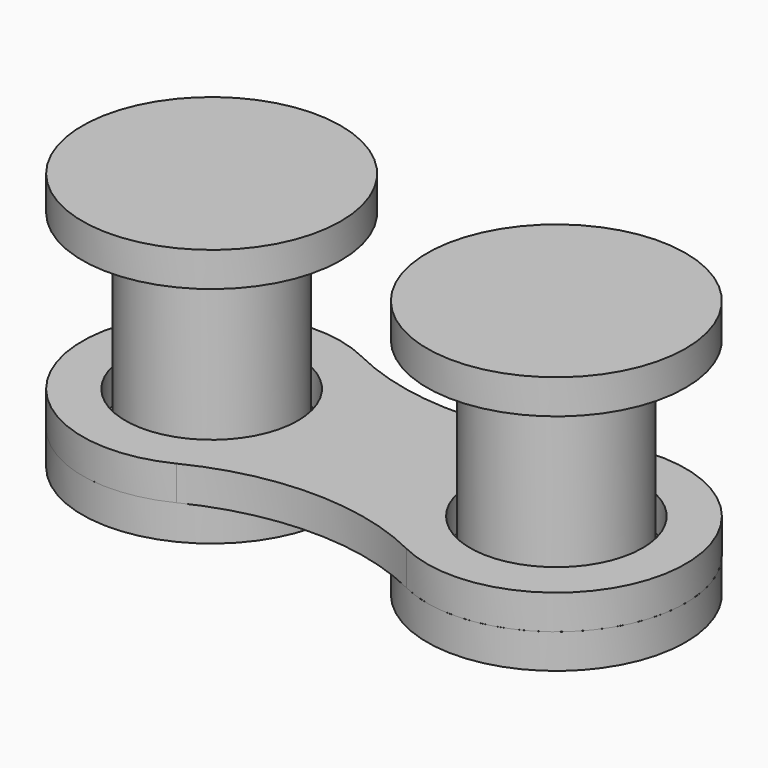
from build123d import *

# Parameters (mm, degrees)
F0_R     = 5
F1_DEPTH = 2
F2_R     = 4.5
F3_DEPTH = 11
F4_R     = 7.5
F5_DEPTH = 2
F6_R     = 7.5
F7_DEPTH = 2


with BuildPart() as f1:
    # F0 (on Top) → F1 (new body)
    with BuildSketch(Plane.XY):
        with BuildLine():
            ThreePointArc((16.6666666667, 6.7185481236), (10, 5.1556443707), (3.3333333333, 6.7185481236))
            ThreePointArc((3.3333333333, 6.7185481236), (-7.5, 0), (3.3333333333, -6.7185481236))
            ThreePointArc((3.3333333333, -6.7185481236), (10, -5.1556443707), (16.6666666667, -6.7185481236))
            ThreePointArc((16.6666666667, -6.7185481236), (27.5, 0), (16.6666666667, 6.7185481236))
        make_face()
        Circle(F0_R, mode=Mode.SUBTRACT)
        with Locations((20, 0)):
            Circle(F0_R, mode=Mode.SUBTRACT)
    extrude(amount=F1_DEPTH)


with BuildPart() as f3:
    # F2 (on Top) → F3 (new body)
    with BuildSketch(Plane.XY):
        Circle(F2_R)
    extrude(amount=F3_DEPTH)

    # F4 (on face) → F5 (join)
    with BuildSketch(Plane.XY.offset(11)):
        Circle(F4_R)
    extrude(amount=F5_DEPTH)

    # F6 (on face) → F7 (join)
    with BuildSketch(Plane(origin=(0, 0, 0), x_dir=(1, 0, 0), z_dir=(0, 0, -1))):
        Circle(F6_R)
    extrude(amount=F7_DEPTH)


with BuildPart() as f3b:
    # F2 (on Top) → F3, piece 2 (new body)
    with BuildSketch(Plane.XY):
        with Locations((20, 0)):
            Circle(F2_R)
    extrude(amount=F3_DEPTH)

    # F4 (on face) → F5, piece 2 (join)
    with BuildSketch(Plane.XY.offset(11)):
        with Locations((20, 0)):
            Circle(F4_R)
    extrude(amount=F5_DEPTH)

    # F6 (on face) → F7, piece 2 (join)
    with BuildSketch(Plane(origin=(0, 0, 0), x_dir=(1, 0, 0), z_dir=(0, 0, -1))):
        with Locations((20, 0)):
            Circle(F6_R)
    extrude(amount=F7_DEPTH)


solid = Compound([f1.part, f3.part, f3b.part])
